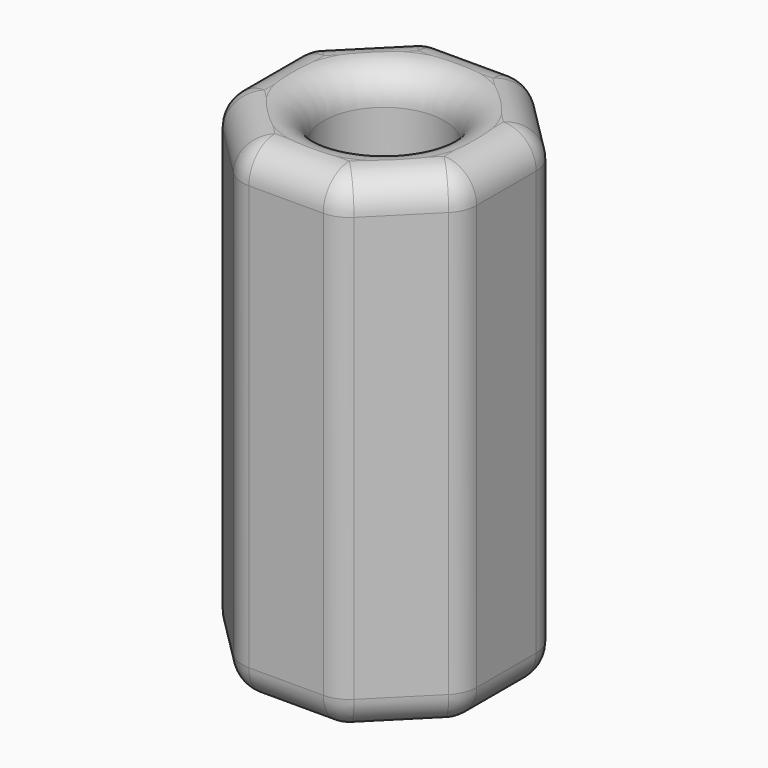
from build123d import *

# Parameters (mm, degrees)
F1_DEPTH      = 30
F2_R          = 3.7
F3_DEPTH      = 15
F4_T3_DEPTH   = 4.5563491861
F4_T5_DEPTH   = 26
F4_T7_DEPTH   = 4.5563491861
F4_T9_DEPTH   = 4.5563491861
F4_T11_DEPTH  = 4.5563491861
F4_T13_DEPTH  = 4.5563491861
F4_T15_DEPTH  = 4.5563491861
F4_T20_DEPTH  = 2
F4_T26_DEPTH  = 2
F4_T32_DEPTH  = 2
F4_T38_DEPTH  = 2
F4_T44_DEPTH  = 2
F4_T50_DEPTH  = 2
F4_T56_DEPTH  = 2
F4_T62_DEPTH  = 2
F4_T68_DEPTH  = 2
F4_T74_DEPTH  = 2
F4_T80_DEPTH  = 2
F4_T86_DEPTH  = 2
F4_T92_DEPTH  = 2
F4_T98_DEPTH  = 2
F4_T104_DEPTH = 2
F4_T110_DEPTH = 2


# Not quite as in the source:
# - a fillet or chamfer that OpenCascade refuses, or shapes differently, is made with other operations: its cross-section is extruded or revolved along the edge and cut away or added


with BuildPart() as f1:
    # F0 (on Top) → F1 (new body)
    with BuildSketch(Plane.XY):
        Polygon((-7.5, 3.1066017178), (-7.5, -3.1066017178), (-3.1066017178, -7.5), (3.1066017178, -7.5), (7.5, -3.1066017178), (7.5, 3.1066017178), (3.1066017178, 7.5), (-3.1066017178, 7.5), align=None)
    extrude(amount=F1_DEPTH)

    # F2 (on face) → F3 (cut)
    with BuildSketch(Plane.XY.offset(30)):
        Circle(F2_R)
    extrude(amount=-F3_DEPTH, mode=Mode.SUBTRACT)

    # F4: fillet of radius 2 on 26 edges, made by hand

    # F4_s1 → F4_t2 (revolve)
    with BuildSketch(Plane.XZ):
        with BuildLine():
            ThreePointArc((3.7, 17), (3.1142135624, 15.5857864376), (1.7, 15))
            Line((1.7, 15), (3.7, 15))
            Line((3.7, 15), (3.7, 17))
        make_face()
    revolve(axis=Axis((0, 0, 15), (0, 0, 1)))

    # F4_s4 → F4_t3 (cut)
    with BuildSketch(Plane(origin=(-1.6109127035, -1.6109127035, 0), x_dir=(0, 0, 1), z_dir=(0.7071067812, 0.7071067812, 0))):
        with BuildLine():
            ThreePointArc((0, 5.5), (0.5857864376, 6.9142135624), (2, 7.5))
            Line((2, 7.5), (0, 7.5))
            Line((0, 7.5), (0, 5.5))
        make_face()
        with BuildLine():
            ThreePointArc((30, 5.5), (29.4142135624, 6.9142135624), (28, 7.5))
            Line((28, 7.5), (30, 7.5))
            Line((30, 7.5), (30, 5.5))
        make_face()
    extrude(amount=F4_T3_DEPTH, mode=Mode.SUBTRACT)

    # F4_s6 → F4_t5 (cut)
    with BuildSketch(Plane.XY.offset(2)):
        with BuildLine():
            ThreePointArc((6.9142135624, -3.6923881554), (7.347759065, -3.0435414578), (7.5, -2.2781745931))
            Line((7.5, -2.2781745931), (7.5, -3.1066017178))
            Line((7.5, -3.1066017178), (6.9142135624, -3.6923881554))
        make_face()
        with BuildLine():
            ThreePointArc((7.5, 2.2781745931), (7.347759065, 3.0435414578), (6.9142135624, 3.6923881554))
            Line((6.9142135624, 3.6923881554), (7.5, 3.1066017178))
            Line((7.5, 3.1066017178), (7.5, 2.2781745931))
        make_face()
        with BuildLine():
            ThreePointArc((-7.5, 2.2781745931), (-7.347759065, 3.0435414578), (-6.9142135624, 3.6923881554))
            Line((-6.9142135624, 3.6923881554), (-7.5, 3.1066017178))
            Line((-7.5, 3.1066017178), (-7.5, 2.2781745931))
        make_face()
        with BuildLine():
            ThreePointArc((-3.6923881554, 6.9142135624), (-3.0435414578, 7.347759065), (-2.2781745931, 7.5))
            Line((-2.2781745931, 7.5), (-3.1066017178, 7.5))
            Line((-3.1066017178, 7.5), (-3.6923881554, 6.9142135624))
        make_face()
        with BuildLine():
            ThreePointArc((-3.6923881554, -6.9142135624), (-3.0435414578, -7.347759065), (-2.2781745931, -7.5))
            Line((-2.2781745931, -7.5), (-3.1066017178, -7.5))
            Line((-3.1066017178, -7.5), (-3.6923881554, -6.9142135624))
        make_face()
        with BuildLine():
            ThreePointArc((-7.5, -2.2781745931), (-7.347759065, -3.0435414578), (-6.9142135624, -3.6923881554))
            Line((-6.9142135624, -3.6923881554), (-7.5, -3.1066017178))
            Line((-7.5, -3.1066017178), (-7.5, -2.2781745931))
        make_face()
        with BuildLine():
            ThreePointArc((2.2781745931, -7.5), (3.0435414578, -7.347759065), (3.6923881554, -6.9142135624))
            Line((3.6923881554, -6.9142135624), (3.1066017178, -7.5))
            Line((3.1066017178, -7.5), (2.2781745931, -7.5))
        make_face()
        with BuildLine():
            ThreePointArc((2.2781745931, 7.5), (3.0435414578, 7.347759065), (3.6923881554, 6.9142135624))
            Line((3.6923881554, 6.9142135624), (3.1066017178, 7.5))
            Line((3.1066017178, 7.5), (2.2781745931, 7.5))
        make_face()
    extrude(amount=F4_T5_DEPTH, mode=Mode.SUBTRACT)

    # F4_s8 → F4_t7 (cut)
    with BuildSketch(Plane.YZ.offset(-2.2781745931)):
        with BuildLine():
            ThreePointArc((-5.5, 0), (-6.9142135624, 0.5857864376), (-7.5, 2))
            Line((-7.5, 2), (-7.5, 0))
            Line((-7.5, 0), (-5.5, 0))
        make_face()
        with BuildLine():
            ThreePointArc((5.5, 0), (6.9142135624, 0.5857864376), (7.5, 2))
            Line((7.5, 2), (7.5, 0))
            Line((7.5, 0), (5.5, 0))
        make_face()
        with BuildLine():
            ThreePointArc((-5.5, 30), (-6.9142135624, 29.4142135624), (-7.5, 28))
            Line((-7.5, 28), (-7.5, 30))
            Line((-7.5, 30), (-5.5, 30))
        make_face()
        with BuildLine():
            ThreePointArc((5.5, 30), (6.9142135624, 29.4142135624), (7.5, 28))
            Line((7.5, 28), (7.5, 30))
            Line((7.5, 30), (5.5, 30))
        make_face()
    extrude(amount=F4_T7_DEPTH, mode=Mode.SUBTRACT)

    # F4_s10 → F4_t9 (cut)
    with BuildSketch(Plane.XZ.offset(-2.2781745931)):
        with BuildLine():
            ThreePointArc((5.5, 30), (6.9142135624, 29.4142135624), (7.5, 28))
            Line((7.5, 28), (7.5, 30))
            Line((7.5, 30), (5.5, 30))
        make_face()
        with BuildLine():
            ThreePointArc((5.5, 0), (6.9142135624, 0.5857864376), (7.5, 2))
            Line((7.5, 2), (7.5, 0))
            Line((7.5, 0), (5.5, 0))
        make_face()
        with BuildLine():
            ThreePointArc((-7.5, 2), (-6.9142135624, 0.5857864376), (-5.5, 0))
            Line((-5.5, 0), (-7.5, 0))
            Line((-7.5, 0), (-7.5, 2))
        make_face()
        with BuildLine():
            ThreePointArc((-7.5, 28), (-6.9142135624, 29.4142135624), (-5.5, 30))
            Line((-5.5, 30), (-7.5, 30))
            Line((-7.5, 30), (-7.5, 28))
        make_face()
    extrude(amount=F4_T9_DEPTH, mode=Mode.SUBTRACT)

    # F4_s12 → F4_t11 (cut)
    with BuildSketch(Plane(origin=(1.6109127035, -1.6109127035, 0), x_dir=(0, 0, 1), z_dir=(-0.7071067812, 0.7071067812, 0))):
        with BuildLine():
            ThreePointArc((0, 5.5), (0.5857864376, 6.9142135624), (2, 7.5))
            Line((2, 7.5), (0, 7.5))
            Line((0, 7.5), (0, 5.5))
        make_face()
        with BuildLine():
            ThreePointArc((30, 5.5), (29.4142135624, 6.9142135624), (28, 7.5))
            Line((28, 7.5), (30, 7.5))
            Line((30, 7.5), (30, 5.5))
        make_face()
    extrude(amount=F4_T11_DEPTH, mode=Mode.SUBTRACT)

    # F4_s14 → F4_t13 (cut)
    with BuildSketch(Plane(origin=(-1.6109127035, 1.6109127035, 0), x_dir=(0, 0, 1), z_dir=(0.7071067812, -0.7071067812, 0))):
        with BuildLine():
            ThreePointArc((2, 7.5), (0.5857864376, 6.9142135624), (0, 5.5))
            Line((0, 5.5), (0, 7.5))
            Line((0, 7.5), (2, 7.5))
        make_face()
        with BuildLine():
            ThreePointArc((28, 7.5), (29.4142135624, 6.9142135624), (30, 5.5))
            Line((30, 5.5), (30, 7.5))
            Line((30, 7.5), (28, 7.5))
        make_face()
    extrude(amount=F4_T13_DEPTH, mode=Mode.SUBTRACT)

    # F4_s16 → F4_t15 (cut)
    with BuildSketch(Plane(origin=(1.6109127035, 1.6109127035, 0), x_dir=(0, 0, 1), z_dir=(-0.7071067812, -0.7071067812, 0))):
        with BuildLine():
            ThreePointArc((28, 7.5), (29.4142135624, 6.9142135624), (30, 5.5))
            Line((30, 5.5), (30, 7.5))
            Line((30, 7.5), (28, 7.5))
        make_face()
        with BuildLine():
            ThreePointArc((2, 7.5), (0.5857864376, 6.9142135624), (0, 5.5))
            Line((0, 5.5), (0, 7.5))
            Line((0, 7.5), (2, 7.5))
        make_face()
    extrude(amount=F4_T15_DEPTH, mode=Mode.SUBTRACT)


with BuildPart() as f4_tool18:
    # F4_s19 → F4_t20 (new body)
    with BuildSketch(Plane.XY.offset(2)):
        Polygon((2.2781745931, -5.5), (2.2781745931, -7.5), (3.1066017178, -7.5), (3.6923881554, -6.9142135624), align=None)
    extrude(amount=-F4_T20_DEPTH)

    # F4_s21 → F4_t22 (revolve, cut)
    with BuildSketch(Plane(origin=(2.2781745931, -5.5, 2), x_dir=(-0.3826834324, 0.9238795325, 0), z_dir=(-0.9238795325, -0.3826834324, 0))):
        with BuildLine():
            ThreePointArc((0, -2), (2, 0), (0, 2))
            Line((0, 2), (0, -2))
        make_face()
    revolve(axis=Axis((2.2781745931, -5.5, 2), (0, 0, -1)), mode=Mode.SUBTRACT)


with BuildPart() as f1_1:
    add(f1.part)

    # F4_t17: cut F4_tool18
    add(f4_tool18.part, mode=Mode.SUBTRACT)


with BuildPart() as f4_tool24:
    # F4_s25 → F4_t26 (new body)
    with BuildSketch(Plane.XY.offset(2)):
        Polygon((5.5, -2.2781745931), (6.9142135624, -3.6923881554), (7.5, -3.1066017178), (7.5, -2.2781745931), align=None)
    extrude(amount=-F4_T26_DEPTH)

    # F4_s27 → F4_t28 (revolve, cut)
    with BuildSketch(Plane(origin=(5.5, -2.2781745931, 2), x_dir=(-0.9238795325, 0.3826834324, 0), z_dir=(-0.3826834324, -0.9238795325, 0))):
        with BuildLine():
            ThreePointArc((0, -2), (2, 0), (0, 2))
            Line((0, 2), (0, -2))
        make_face()
    revolve(axis=Axis((5.5, -2.2781745931, 2), (0, 0, -1)), mode=Mode.SUBTRACT)


with BuildPart() as f1_2:
    add(f1_1.part)

    # F4_t23: cut F4_tool24
    add(f4_tool24.part, mode=Mode.SUBTRACT)


with BuildPart() as f4_tool30:
    # F4_s31 → F4_t32 (new body)
    with BuildSketch(Plane.XY.offset(28)):
        Polygon((5.5, -2.2781745931), (6.9142135624, -3.6923881554), (7.5, -3.1066017178), (7.5, -2.2781745931), align=None)
    extrude(amount=F4_T32_DEPTH)

    # F4_s33 → F4_t34 (revolve, cut)
    with BuildSketch(Plane(origin=(5.5, -2.2781745931, 28), x_dir=(-0.9238795325, 0.3826834324, 0), z_dir=(0.3826834324, 0.9238795325, 0))):
        with BuildLine():
            ThreePointArc((0, -2), (2, 0), (0, 2))
            Line((0, 2), (0, -2))
        make_face()
    revolve(axis=Axis((5.5, -2.2781745931, 28), (0, 0, 1)), mode=Mode.SUBTRACT)


with BuildPart() as f1_3:
    add(f1_2.part)

    # F4_t29: cut F4_tool30
    add(f4_tool30.part, mode=Mode.SUBTRACT)


with BuildPart() as f4_tool36:
    # F4_s37 → F4_t38 (new body)
    with BuildSketch(Plane.XY.offset(2)):
        Polygon((5.5, 2.2781745931), (7.5, 2.2781745931), (7.5, 3.1066017178), (6.9142135624, 3.6923881554), align=None)
    extrude(amount=-F4_T38_DEPTH)

    # F4_s39 → F4_t40 (revolve, cut)
    with BuildSketch(Plane(origin=(5.5, 2.2781745931, 2), x_dir=(-0.9238795325, -0.3826834324, 0), z_dir=(0.3826834324, -0.9238795325, 0))):
        with BuildLine():
            ThreePointArc((0, -2), (2, 0), (0, 2))
            Line((0, 2), (0, -2))
        make_face()
    revolve(axis=Axis((5.5, 2.2781745931, 2), (0, 0, -1)), mode=Mode.SUBTRACT)


with BuildPart() as f1_4:
    add(f1_3.part)

    # F4_t35: cut F4_tool36
    add(f4_tool36.part, mode=Mode.SUBTRACT)


with BuildPart() as f4_tool42:
    # F4_s43 → F4_t44 (new body)
    with BuildSketch(Plane.XY.offset(28)):
        Polygon((5.5, 2.2781745931), (7.5, 2.2781745931), (7.5, 3.1066017178), (6.9142135624, 3.6923881554), align=None)
    extrude(amount=F4_T44_DEPTH)

    # F4_s45 → F4_t46 (revolve, cut)
    with BuildSketch(Plane(origin=(5.5, 2.2781745931, 28), x_dir=(-0.9238795325, -0.3826834324, 0), z_dir=(-0.3826834324, 0.9238795325, 0))):
        with BuildLine():
            ThreePointArc((0, -2), (2, 0), (0, 2))
            Line((0, 2), (0, -2))
        make_face()
    revolve(axis=Axis((5.5, 2.2781745931, 28), (0, 0, 1)), mode=Mode.SUBTRACT)


with BuildPart() as f1_5:
    add(f1_4.part)

    # F4_t41: cut F4_tool42
    add(f4_tool42.part, mode=Mode.SUBTRACT)


with BuildPart() as f4_tool48:
    # F4_s49 → F4_t50 (new body)
    with BuildSketch(Plane.XY.offset(2)):
        Polygon((-2.2781745931, -5.5), (-2.2781745931, -7.5), (-3.1066017178, -7.5), (-3.6923881554, -6.9142135624), align=None)
    extrude(amount=-F4_T50_DEPTH)

    # F4_s51 → F4_t52 (revolve, cut)
    with BuildSketch(Plane(origin=(-2.2781745931, -5.5, 2), x_dir=(0.3826834324, 0.9238795325, 0), z_dir=(-0.9238795325, 0.3826834324, 0))):
        with BuildLine():
            ThreePointArc((0, -2), (2, 0), (0, 2))
            Line((0, 2), (0, -2))
        make_face()
    revolve(axis=Axis((-2.2781745931, -5.5, 2), (0, 0, -1)), mode=Mode.SUBTRACT)


with BuildPart() as f1_6:
    add(f1_5.part)

    # F4_t47: cut F4_tool48
    add(f4_tool48.part, mode=Mode.SUBTRACT)


with BuildPart() as f4_tool54:
    # F4_s55 → F4_t56 (new body)
    with BuildSketch(Plane.XY.offset(2)):
        Polygon((2.2781745931, 5.5), (2.2781745931, 7.5), (3.1066017178, 7.5), (3.6923881554, 6.9142135624), align=None)
    extrude(amount=-F4_T56_DEPTH)

    # F4_s57 → F4_t58 (revolve, cut)
    with BuildSketch(Plane(origin=(2.2781745931, 5.5, 2), x_dir=(-0.3826834324, -0.9238795325, 0), z_dir=(0.9238795325, -0.3826834324, 0))):
        with BuildLine():
            ThreePointArc((0, -2), (2, 0), (0, 2))
            Line((0, 2), (0, -2))
        make_face()
    revolve(axis=Axis((2.2781745931, 5.5, 2), (0, 0, -1)), mode=Mode.SUBTRACT)


with BuildPart() as f1_7:
    add(f1_6.part)

    # F4_t53: cut F4_tool54
    add(f4_tool54.part, mode=Mode.SUBTRACT)


with BuildPart() as f4_tool60:
    # F4_s61 → F4_t62 (new body)
    with BuildSketch(Plane.XY.offset(2)):
        Polygon((-2.2781745931, 5.5), (-2.2781745931, 7.5), (-3.1066017178, 7.5), (-3.6923881554, 6.9142135624), align=None)
    extrude(amount=-F4_T62_DEPTH)

    # F4_s63 → F4_t64 (revolve, cut)
    with BuildSketch(Plane(origin=(-2.2781745931, 5.5, 2), x_dir=(0.3826834324, -0.9238795325, 0), z_dir=(0.9238795325, 0.3826834324, 0))):
        with BuildLine():
            ThreePointArc((0, -2), (2, 0), (0, 2))
            Line((0, 2), (0, -2))
        make_face()
    revolve(axis=Axis((-2.2781745931, 5.5, 2), (0, 0, -1)), mode=Mode.SUBTRACT)


with BuildPart() as f1_8:
    add(f1_7.part)

    # F4_t59: cut F4_tool60
    add(f4_tool60.part, mode=Mode.SUBTRACT)


with BuildPart() as f4_tool66:
    # F4_s67 → F4_t68 (new body)
    with BuildSketch(Plane.XY.offset(2)):
        Polygon((-5.5, -2.2781745931), (-7.5, -2.2781745931), (-7.5, -3.1066017178), (-6.9142135624, -3.6923881554), align=None)
    extrude(amount=-F4_T68_DEPTH)

    # F4_s69 → F4_t70 (revolve, cut)
    with BuildSketch(Plane(origin=(-5.5, -2.2781745931, 2), x_dir=(0.9238795325, 0.3826834324, 0), z_dir=(-0.3826834324, 0.9238795325, 0))):
        with BuildLine():
            ThreePointArc((0, -2), (2, 0), (0, 2))
            Line((0, 2), (0, -2))
        make_face()
    revolve(axis=Axis((-5.5, -2.2781745931, 2), (0, 0, -1)), mode=Mode.SUBTRACT)


with BuildPart() as f1_9:
    add(f1_8.part)

    # F4_t65: cut F4_tool66
    add(f4_tool66.part, mode=Mode.SUBTRACT)


with BuildPart() as f4_tool72:
    # F4_s73 → F4_t74 (new body)
    with BuildSketch(Plane.XY.offset(2)):
        Polygon((-5.5, 2.2781745931), (-7.5, 2.2781745931), (-7.5, 3.1066017178), (-6.9142135624, 3.6923881554), align=None)
    extrude(amount=-F4_T74_DEPTH)

    # F4_s75 → F4_t76 (revolve, cut)
    with BuildSketch(Plane(origin=(-5.5, 2.2781745931, 2), x_dir=(0.9238795325, -0.3826834324, 0), z_dir=(0.3826834324, 0.9238795325, 0))):
        with BuildLine():
            ThreePointArc((0, -2), (2, 0), (0, 2))
            Line((0, 2), (0, -2))
        make_face()
    revolve(axis=Axis((-5.5, 2.2781745931, 2), (0, 0, -1)), mode=Mode.SUBTRACT)


with BuildPart() as f1_10:
    add(f1_9.part)

    # F4_t71: cut F4_tool72
    add(f4_tool72.part, mode=Mode.SUBTRACT)


with BuildPart() as f4_tool78:
    # F4_s79 → F4_t80 (new body)
    with BuildSketch(Plane.XY.offset(28)):
        Polygon((-5.5, 2.2781745931), (-7.5, 2.2781745931), (-7.5, 3.1066017178), (-6.9142135624, 3.6923881554), align=None)
    extrude(amount=F4_T80_DEPTH)

    # F4_s81 → F4_t82 (revolve, cut)
    with BuildSketch(Plane(origin=(-5.5, 2.2781745931, 28), x_dir=(0.9238795325, -0.3826834324, 0), z_dir=(-0.3826834324, -0.9238795325, 0))):
        with BuildLine():
            ThreePointArc((0, -2), (2, 0), (0, 2))
            Line((0, 2), (0, -2))
        make_face()
    revolve(axis=Axis((-5.5, 2.2781745931, 28), (0, 0, 1)), mode=Mode.SUBTRACT)


with BuildPart() as f1_11:
    add(f1_10.part)

    # F4_t77: cut F4_tool78
    add(f4_tool78.part, mode=Mode.SUBTRACT)


with BuildPart() as f4_tool84:
    # F4_s85 → F4_t86 (new body)
    with BuildSketch(Plane.XY.offset(28)):
        Polygon((-2.2781745931, 5.5), (-2.2781745931, 7.5), (-3.1066017178, 7.5), (-3.6923881554, 6.9142135624), align=None)
    extrude(amount=F4_T86_DEPTH)

    # F4_s87 → F4_t88 (revolve, cut)
    with BuildSketch(Plane(origin=(-2.2781745931, 5.5, 28), x_dir=(0.3826834324, -0.9238795325, 0), z_dir=(-0.9238795325, -0.3826834324, 0))):
        with BuildLine():
            ThreePointArc((0, -2), (2, 0), (0, 2))
            Line((0, 2), (0, -2))
        make_face()
    revolve(axis=Axis((-2.2781745931, 5.5, 28), (0, 0, 1)), mode=Mode.SUBTRACT)


with BuildPart() as f1_12:
    add(f1_11.part)

    # F4_t83: cut F4_tool84
    add(f4_tool84.part, mode=Mode.SUBTRACT)


with BuildPart() as f4_tool90:
    # F4_s91 → F4_t92 (new body)
    with BuildSketch(Plane.XY.offset(28)):
        Polygon((-2.2781745931, -5.5), (-2.2781745931, -7.5), (-3.1066017178, -7.5), (-3.6923881554, -6.9142135624), align=None)
    extrude(amount=F4_T92_DEPTH)

    # F4_s93 → F4_t94 (revolve, cut)
    with BuildSketch(Plane(origin=(-2.2781745931, -5.5, 28), x_dir=(0.3826834324, 0.9238795325, 0), z_dir=(0.9238795325, -0.3826834324, 0))):
        with BuildLine():
            ThreePointArc((0, -2), (2, 0), (0, 2))
            Line((0, 2), (0, -2))
        make_face()
    revolve(axis=Axis((-2.2781745931, -5.5, 28), (0, 0, 1)), mode=Mode.SUBTRACT)


with BuildPart() as f1_13:
    add(f1_12.part)

    # F4_t89: cut F4_tool90
    add(f4_tool90.part, mode=Mode.SUBTRACT)


with BuildPart() as f4_tool96:
    # F4_s97 → F4_t98 (new body)
    with BuildSketch(Plane.XY.offset(28)):
        Polygon((-5.5, -2.2781745931), (-7.5, -2.2781745931), (-7.5, -3.1066017178), (-6.9142135624, -3.6923881554), align=None)
    extrude(amount=F4_T98_DEPTH)

    # F4_s99 → F4_t100 (revolve, cut)
    with BuildSketch(Plane(origin=(-5.5, -2.2781745931, 28), x_dir=(0.9238795325, 0.3826834324, 0), z_dir=(0.3826834324, -0.9238795325, 0))):
        with BuildLine():
            ThreePointArc((0, -2), (2, 0), (0, 2))
            Line((0, 2), (0, -2))
        make_face()
    revolve(axis=Axis((-5.5, -2.2781745931, 28), (0, 0, 1)), mode=Mode.SUBTRACT)


with BuildPart() as f1_14:
    add(f1_13.part)

    # F4_t95: cut F4_tool96
    add(f4_tool96.part, mode=Mode.SUBTRACT)


with BuildPart() as f4_tool102:
    # F4_s103 → F4_t104 (new body)
    with BuildSketch(Plane.XY.offset(28)):
        Polygon((2.2781745931, -5.5), (2.2781745931, -7.5), (3.1066017178, -7.5), (3.6923881554, -6.9142135624), align=None)
    extrude(amount=F4_T104_DEPTH)

    # F4_s105 → F4_t106 (revolve, cut)
    with BuildSketch(Plane(origin=(2.2781745931, -5.5, 28), x_dir=(-0.3826834324, 0.9238795325, 0), z_dir=(0.9238795325, 0.3826834324, 0))):
        with BuildLine():
            ThreePointArc((0, -2), (2, 0), (0, 2))
            Line((0, 2), (0, -2))
        make_face()
    revolve(axis=Axis((2.2781745931, -5.5, 28), (0, 0, 1)), mode=Mode.SUBTRACT)


with BuildPart() as f1_15:
    add(f1_14.part)

    # F4_t101: cut F4_tool102
    add(f4_tool102.part, mode=Mode.SUBTRACT)


with BuildPart() as f4_tool108:
    # F4_s109 → F4_t110 (new body)
    with BuildSketch(Plane.XY.offset(28)):
        Polygon((2.2781745931, 5.5), (2.2781745931, 7.5), (3.1066017178, 7.5), (3.6923881554, 6.9142135624), align=None)
    extrude(amount=F4_T110_DEPTH)

    # F4_s111 → F4_t112 (revolve, cut)
    with BuildSketch(Plane(origin=(2.2781745931, 5.5, 28), x_dir=(-0.3826834324, -0.9238795325, 0), z_dir=(-0.9238795325, 0.3826834324, 0))):
        with BuildLine():
            ThreePointArc((0, -2), (2, 0), (0, 2))
            Line((0, 2), (0, -2))
        make_face()
    revolve(axis=Axis((2.2781745931, 5.5, 28), (0, 0, 1)), mode=Mode.SUBTRACT)


with BuildPart() as f1_16:
    add(f1_15.part)

    # F4_t107: cut F4_tool108
    add(f4_tool108.part, mode=Mode.SUBTRACT)

    # F4_s113 → F4_t114 (revolve, cut)
    with BuildSketch(Plane.XZ):
        with BuildLine():
            ThreePointArc((5.7, 30), (4.2857864376, 29.4142135624), (3.7, 28))
            Line((3.7, 28), (3.7, 30))
            Line((3.7, 30), (5.7, 30))
        make_face()
    revolve(axis=Axis((0, 0, 30), (0, 0, 1)), mode=Mode.SUBTRACT)


solid = f1_16.part
